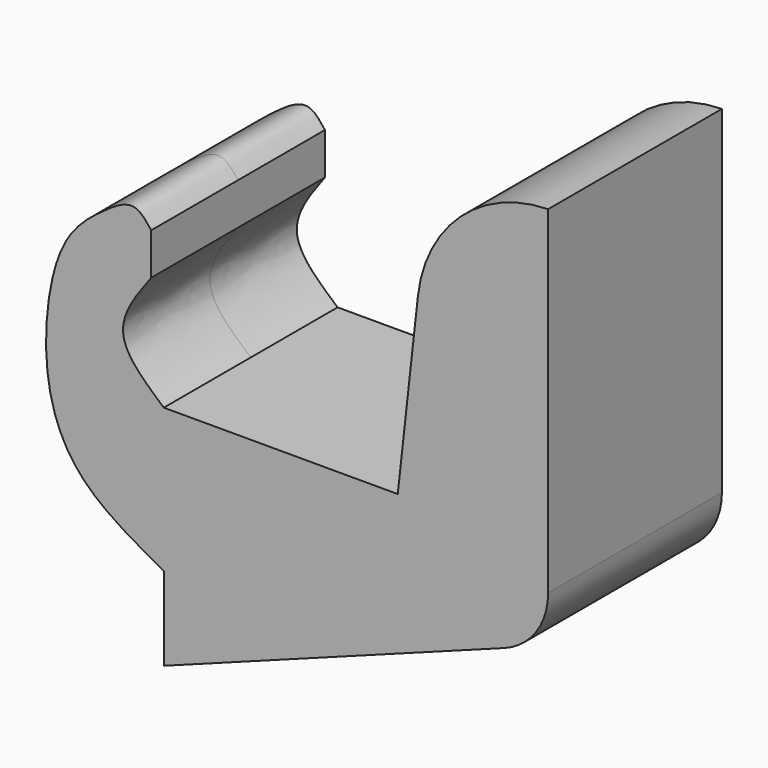
from build123d import *

# Parameters (mm, degrees)
F1_DEPTH    = 6.5
F2_T1_DEPTH = 48.7796937487
F3_R        = 4


# Not quite as in the source:
# - a fillet or chamfer that OpenCascade refuses, or shapes differently, is made with other operations: its cross-section is extruded or revolved along the edge and cut away or added


with BuildPart() as f1:
    # F0 (on Front) → F1 (new body, symmetric)
    with BuildSketch(Plane.XZ):
        with BuildLine():
            Line((0, 0), (-14, 0))
            add(Edge.make_bspline(
                [(-14.753227005, 6.6), (-15.6505771516, 5.402281958), (-17.4537159579, 2.9955827572), (-15.1548248478, 1.0016380744), (-14, 0)],
                knots=[0, 0, 0, 0, 0.4976600489, 1, 1, 1, 1], degree=3))
            Line((-14.753227005, 6.6), (-14.753227005, 9.1))
            add(Edge.make_bspline(
                [(-14.753227005, 9.1), (-15.0782830968, 9.5217558402), (-15.8019667592, 10.4607255098), (-17.9577835755, 8.9859803429), (-20.5635971664, 6.8288464563), (-21.5233314219, -0.162172448), (-19.5302154879, -5.5960603901), (-15.8730160291, -7.5826025673), (-14, -8.6)],
                knots=[0, 0, 0, 0, 0.1000363237, 0.2227143405, 0.3768740844, 0.5944901084, 0.7923201796, 1, 1, 1, 1], degree=3))
            Line((-14, -8.6), (-14, -13.6))
            Line((-14, -13.6), (9, -5.0644312273))
            Line((9, -5.0644312273), (9, 17.9355687727))
            Line((9, 17.9355687727), (2, 17.9355687727))
            Line((2, 17.9355687727), (0.7464859836, 6.6943253484))
            Line((0.7464859836, 6.6943253484), (0.3732429918, 3.3471626742))
            Line((0.3732429918, 3.3471626742), (0, 0))
        make_face()
    extrude(amount=F1_DEPTH, both=True)

    # F2: fillet of radius 8 on 1 edges, made by hand

    # F2_s2 → F2_t1 (cut)
    with BuildSketch(Plane.XZ.offset(-24.3898468744)):
        with BuildLine():
            ThreePointArc((1.2069547277, 10.8237097622), (3.7649807454, 15.8463394269), (9, 17.9355687727))
            Line((9, 17.9355687727), (2, 17.9355687727))
            Line((2, 17.9355687727), (1.2069547277, 10.8237097622))
        make_face()
    extrude(amount=F2_T1_DEPTH, mode=Mode.SUBTRACT)

    # F3
    f3_edges = [f1.edges().sort_by_distance(p)[0] for p in [
        (9, 0, -5.064431),
    ]]
    fillet(f3_edges, radius=F3_R)


solid = f1.part
